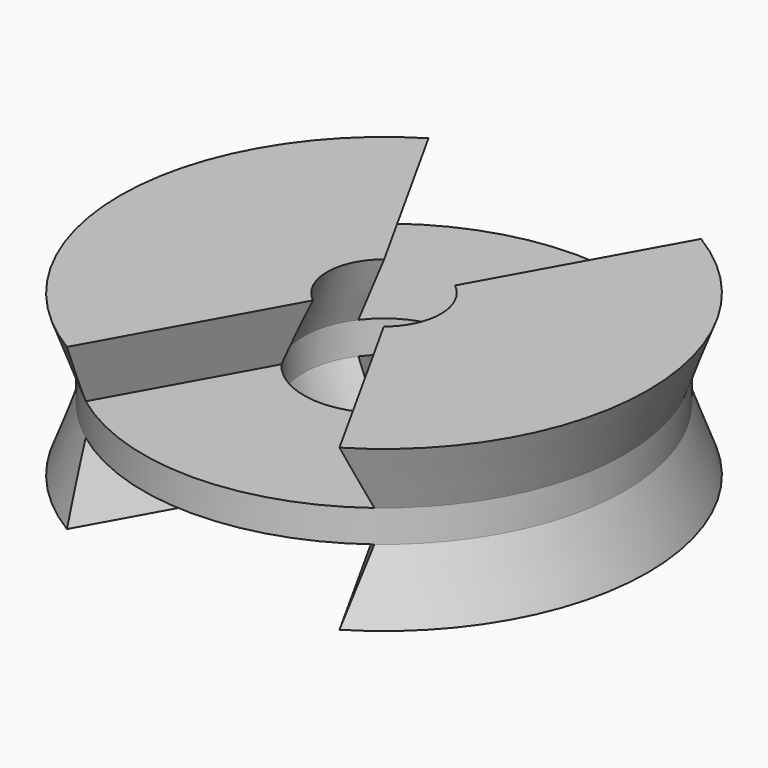
from build123d import *

# Parameters (mm, degrees)
F0_R                     = 15
F0_R_2                   = 5
F1_DEPTH                 = 2
F3_DEPTH                 = 4
DRAFT_F3_DRAFTED_ANGLE   = -20
DRAFT_F3_2_DRAFTED_ANGLE = -20
F5_DEPTH                 = 4
DRAFT_F5_DRAFTED_ANGLE   = -20
DRAFT_F5_2_DRAFTED_ANGLE = -20


# Not quite as in the source:
# - an extrude with a draft is written as a straight extrude whose walls are then drafted


with BuildPart() as f1:
    # F0 (on Top) → F1 (new body)
    with BuildSketch(Plane.XY):
        Circle(F0_R)
        Circle(F0_R_2, mode=Mode.SUBTRACT)
    extrude(amount=F1_DEPTH)


with BuildPart() as f3_drafted:
    # F2 (on face) → F3 (new body)
    with BuildSketch(Plane.XY.offset(2)):
        with BuildLine():
            ThreePointArc((-4, -3), (-5, 0), (-4, 3))
            Line((-4, 3), (-9, 12))
            ThreePointArc((-9, 12), (-15, 0), (-9, -12))
            Line((-9, -12), (-4, -3))
        make_face()
    extrude(amount=F3_DEPTH)

    # draft_F3_drafted
    draft_f3_drafted_walls = [f3_drafted.faces().sort_by_distance(p)[0] for p in [
        (-6.5, -7.5, 4.6666666667),
        (-5, 0, 4.6666666667),
        (-6.5, 7.5, 4.6666666667),
        (-15, 0, 4.6666666667),
    ]]
    draft(draft_f3_drafted_walls, neutral_plane=Plane.XY.offset(2), angle=DRAFT_F3_DRAFTED_ANGLE)


with BuildPart() as f1_1:
    add(f1.part)

    # join_F3_drafted: union F3_drafted
    add(f3_drafted.part)


with BuildPart() as f3_2_drafted:
    # F2 (on face) → F3, piece 2 (new body)
    with BuildSketch(Plane.XY.offset(2)):
        with BuildLine():
            Line((9, 12), (4, 3))
            ThreePointArc((4, 3), (4.7434164903, 1.5811388301), (5, 0))
            ThreePointArc((5, 0), (4.7434164903, -1.5811388301), (4, -3))
            Line((4, -3), (9, -12))
            ThreePointArc((9, -12), (13.416407865, -6.7082039325), (15, 0))
            ThreePointArc((15, 0), (13.416407865, 6.7082039325), (9, 12))
        make_face()
    extrude(amount=F3_DEPTH)

    # draft_F3_2_drafted
    draft_f3_2_drafted_walls = [f3_2_drafted.faces().sort_by_distance(p)[0] for p in [
        (15, 0, 4.6666666667),
        (5, 0, 4.6666666667),
        (6.5, -7.5, 4.6666666667),
        (6.5, 7.5, 4.6666666667),
    ]]
    draft(draft_f3_2_drafted_walls, neutral_plane=Plane.XY.offset(2), angle=DRAFT_F3_2_DRAFTED_ANGLE)


with BuildPart() as f1_2:
    add(f1_1.part)

    # join_F3_2_drafted: union F3_2_drafted
    add(f3_2_drafted.part)


with BuildPart() as f5_drafted:
    # F4 (on face) → F5 (new body)
    with BuildSketch(Plane(origin=(0, 0, 0), x_dir=(1, 0, 0), z_dir=(0, 0, -1))):
        with BuildLine():
            ThreePointArc((-4, -3), (-5, 0), (-4, 3))
            Line((-4, 3), (-9, 12))
            ThreePointArc((-9, 12), (-15, 0), (-9, -12))
            Line((-9, -12), (-4, -3))
        make_face()
    extrude(amount=F5_DEPTH)

    # draft_F5_drafted
    draft_f5_drafted_walls = [f5_drafted.faces().sort_by_distance(p)[0] for p in [
        (-6.5, 7.5, -2.6666666667),
        (-5, 0, -2.6666666667),
        (-6.5, -7.5, -2.6666666667),
        (-15, 0, -2.6666666667),
    ]]
    draft(draft_f5_drafted_walls, neutral_plane=Plane(origin=(0, 0, 0), x_dir=(1, 0, 0), z_dir=(0, 0, -1)), angle=DRAFT_F5_DRAFTED_ANGLE)


with BuildPart() as f1_3:
    add(f1_2.part)

    # join_F5_drafted: union F5_drafted
    add(f5_drafted.part)


with BuildPart() as f5_2_drafted:
    # F4 (on face) → F5, piece 2 (new body)
    with BuildSketch(Plane(origin=(0, 0, 0), x_dir=(1, 0, 0), z_dir=(0, 0, -1))):
        with BuildLine():
            Line((9, 12), (4, 3))
            ThreePointArc((4, 3), (4.7434164903, 1.5811388301), (5, 0))
            ThreePointArc((5, 0), (4.7434164903, -1.5811388301), (4, -3))
            Line((4, -3), (9, -12))
            ThreePointArc((9, -12), (13.416407865, -6.7082039325), (15, 0))
            ThreePointArc((15, 0), (13.416407865, 6.7082039325), (9, 12))
        make_face()
    extrude(amount=F5_DEPTH)

    # draft_F5_2_drafted
    draft_f5_2_drafted_walls = [f5_2_drafted.faces().sort_by_distance(p)[0] for p in [
        (15, 0, -2.6666666667),
        (5, 0, -2.6666666667),
        (6.5, 7.5, -2.6666666667),
        (6.5, -7.5, -2.6666666667),
    ]]
    draft(draft_f5_2_drafted_walls, neutral_plane=Plane(origin=(0, 0, 0), x_dir=(1, 0, 0), z_dir=(0, 0, -1)), angle=DRAFT_F5_2_DRAFTED_ANGLE)


with BuildPart() as f1_4:
    add(f1_3.part)

    # join_F5_2_drafted: union F5_2_drafted
    add(f5_2_drafted.part)


solid = f1_4.part
